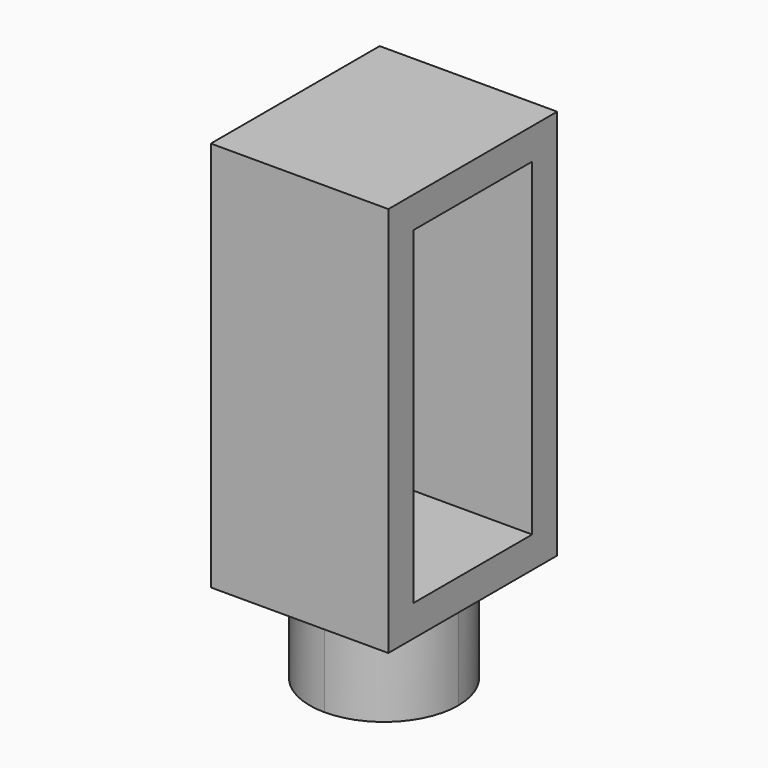
from build123d import *

# Parameters (mm, degrees)
F0_R     = 3.5
F1_DEPTH = 2
F2_DEPTH = 23
F3_W     = 11.3556964174
F3_H     = 13.5
F4_DEPTH = 2
F5_DEPTH = 6


with BuildPart() as f1:
    # F0 (on Top) → F1 (new body)
    with BuildSketch(Plane.XY):
        Polygon((-4.6443035826, -6.75), (-4.6443035826, -4.75), (-10.3221517913, -4.75), (-16, -4.75), (-16, -6.75), align=None)
        with BuildLine():
            Line((-10.3221517913, -4.75), (-4.6443035826, -4.75))
            Line((-4.6443035826, -4.75), (-4.6443035826, 4.75))
            Line((-4.6443035826, 4.75), (-10.3221517821, 4.75))
            ThreePointArc((-10.3221517821, 4.75), (-6.9633945774, 3.3587572074), (-5.5721517913, 0))
            ThreePointArc((-5.5721517913, 0), (-6.9633945807, -3.3587572106), (-10.3221517913, -4.75))
        make_face()
        with BuildLine():
            Line((-16, -4.75), (-10.3221517913, -4.75))
            ThreePointArc((-10.3221517913, -4.75), (-15.0721517913, 4.6e-09), (-10.3221517821, 4.75))
            Line((-10.3221517821, 4.75), (-16, 4.75))
            Line((-16, 4.75), (-16, -4.75))
        make_face()
        with BuildLine():
            ThreePointArc((-10.3221517821, 4.75), (-15.0721517913, 4.6e-09), (-10.3221517913, -4.75))
            ThreePointArc((-10.3221517913, -4.75), (-6.9633945807, -3.3587572106), (-5.5721517913, 0))
            ThreePointArc((-5.5721517913, 0), (-6.9633945774, 3.3587572074), (-10.3221517821, 4.75))
        make_face()
        with Locations((-10.3221517913, 0)):
            Circle(F0_R, mode=Mode.SUBTRACT)
        Polygon((-10.3221517821, 4.75), (-4.6443035826, 4.75), (-4.6443035826, 6.75), (-16, 6.75), (-16, 4.75), align=None)
        with Locations((-10.3221517913, 0)):
            Circle(F0_R)
    extrude(amount=F1_DEPTH)

    # F0 (on Top) → F2 (join)
    with BuildSketch(Plane.XY):
        Polygon((-10.3221517821, 4.75), (-4.6443035826, 4.75), (-4.6443035826, 6.75), (-16, 6.75), (-16, 4.75), align=None)
        Polygon((-4.6443035826, -6.75), (-4.6443035826, -4.75), (-10.3221517913, -4.75), (-16, -4.75), (-16, -6.75), align=None)
    extrude(amount=F2_DEPTH)

    # F3 (on face) → F4 (join)
    with BuildSketch(Plane.XY.offset(23)):
        with Locations((-10.3221517913, 0)):
            Rectangle(F3_W, F3_H)
    extrude(amount=F4_DEPTH)

    # F0 (on Top) → F5 (join)
    with BuildSketch(Plane.XY):
        with BuildLine():
            ThreePointArc((-10.3221517821, 4.75), (-15.0721517913, 4.6e-09), (-10.3221517913, -4.75))
            ThreePointArc((-10.3221517913, -4.75), (-6.9633945807, -3.3587572106), (-5.5721517913, 0))
            ThreePointArc((-5.5721517913, 0), (-6.9633945774, 3.3587572074), (-10.3221517821, 4.75))
        make_face()
        with Locations((-10.3221517913, 0)):
            Circle(F0_R, mode=Mode.SUBTRACT)
    extrude(amount=-F5_DEPTH)


solid = f1.part
